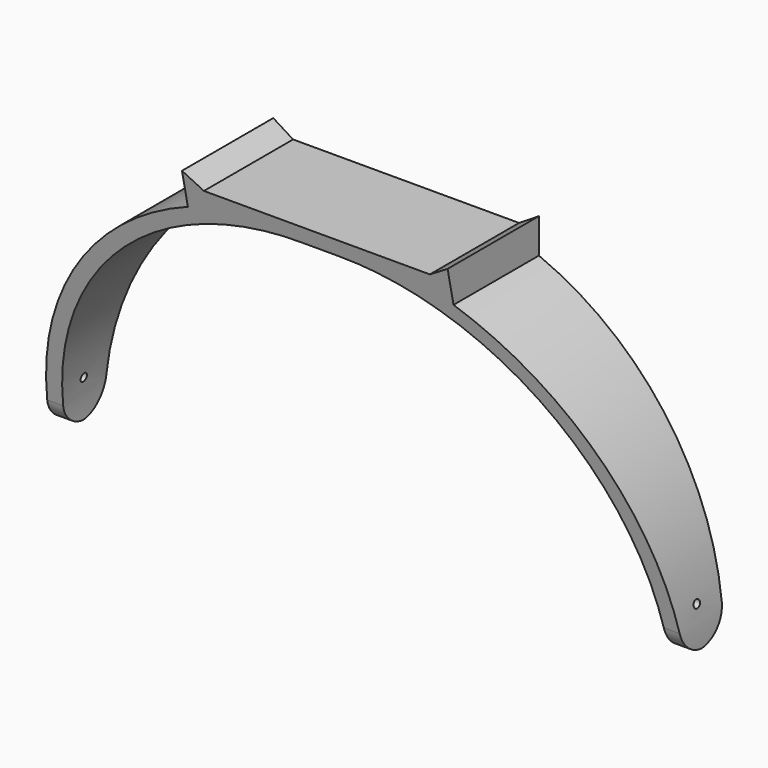
from build123d import *

# Parameters (mm, degrees)
F1_DEPTH      = 25.4
F3_DEPTH      = 40.641
F3_DEPTH_BACK = 40.641
F4_R          = 0.508
F5_DEPTH      = 40.641
F5_DEPTH_BACK = 40.641
F6_T1_DEPTH   = 17.4583858324
F6_T3_DEPTH   = 21.082
F6_T5_DEPTH   = 21.082
F6_T7_DEPTH   = 17.4583858324


# Not quite as in the source:
# - a fillet or chamfer that OpenCascade refuses, or shapes differently, is made with other operations: its cross-section is extruded or revolved along the edge and cut away or added


with BuildPart() as f1:
    # F0 (on Front) → F1 (new body)
    with BuildSketch(Plane.XZ):
        with BuildLine():
            Line((2.54, 0), (0, 0))
            Line((0, 0), (-2.54, 0))
            Line((-2.54, 0), (-14.478, 0))
            Line((-14.478, 0), (-17.018, 0))
            Line((-17.018, 0), (-17.018, -2.8580148686))
            ThreePointArc((-17.018, -2.8580148686), (-34.1882369177, -16.8868177776), (-40.64, -38.1))
            Line((-40.64, -38.1), (-38.608, -38.1))
            ThreePointArc((-38.608, -38.1), (-28.0439273838, -12.5960726162), (-2.54, -2.032))
            Line((-2.54, -2.032), (0, -2.032))
            Line((0, -2.032), (2.54, -2.032))
            ThreePointArc((2.54, -2.032), (28.0439273838, -12.5960726162), (38.608, -38.1))
            Line((38.608, -38.1), (40.64, -38.1))
            ThreePointArc((40.64, -38.1), (34.1882369177, -16.8868177776), (17.018, -2.8580148686))
            Line((17.018, -2.8580148686), (17.018, 0))
            Line((17.018, 0), (14.478, 0))
            Line((14.478, 0), (2.54, 0))
        make_face()
        Polygon((-17.018, 0), (-14.478, 0), (-17.018, 1.5875), align=None)
        Polygon((17.018, 1.5875), (14.478, 0), (17.018, 0), align=None)
    extrude(amount=F1_DEPTH)

    # F2 (on Right) → F3 (cut, two sides)
    with BuildSketch(Plane.YZ) as f3_sk:
        Polygon((-30.48, -50.8), (-3.4853166679, -50.8), (-30.48, 76.2), align=None)
    extrude(amount=-F3_DEPTH, mode=Mode.SUBTRACT)
    extrude(f3_sk.sketch, amount=F3_DEPTH_BACK, mode=Mode.SUBTRACT)

    # F4 (on Right) → F5 (cut, two sides)
    with BuildSketch(Plane.YZ) as f5_sk:
        with Locations((-3.81, -33.02)):
            Circle(F4_R)
    extrude(amount=-F5_DEPTH, mode=Mode.SUBTRACT)
    extrude(f5_sk.sketch, amount=F5_DEPTH_BACK, mode=Mode.SUBTRACT)

    # F6: fillet of radius 3.81 on 4 edges, made by hand

    # F6_s2 → F6_t1 (cut)
    with BuildSketch(Plane.YZ.offset(30.8948070838)):
        with BuildLine():
            ThreePointArc((-6.8262501934, -35.082143542), (-5.4972185245, -37.2509261132), (-3.0995078346, -38.1))
            Line((-3.0995078346, -38.1), (-6.1847850011, -38.1))
            Line((-6.1847850011, -38.1), (-6.8262501934, -35.082143542))
        make_face()
    extrude(amount=F6_T1_DEPTH, mode=Mode.SUBTRACT)

    # F6_s4 → F6_t3 (cut)
    with BuildSketch(Plane.YZ.offset(29.083)):
        with BuildLine():
            ThreePointArc((0, -34.29), (-1.1159231637, -36.9840768363), (-3.81, -38.1))
            Line((-3.81, -38.1), (0, -38.1))
            Line((0, -38.1), (0, -34.29))
        make_face()
    extrude(amount=F6_T3_DEPTH, mode=Mode.SUBTRACT)

    # F6_s6 → F6_t5 (cut)
    with BuildSketch(Plane.YZ.offset(-50.165)):
        with BuildLine():
            ThreePointArc((0, -34.29), (-1.1159231637, -36.9840768363), (-3.81, -38.1))
            Line((-3.81, -38.1), (0, -38.1))
            Line((0, -38.1), (0, -34.29))
        make_face()
    extrude(amount=F6_T5_DEPTH, mode=Mode.SUBTRACT)

    # F6_s8 → F6_t7 (cut)
    with BuildSketch(Plane.YZ.offset(-48.3531929162)):
        with BuildLine():
            ThreePointArc((-6.8262501934, -35.082143542), (-5.4972185245, -37.2509261132), (-3.0995078346, -38.1))
            Line((-3.0995078346, -38.1), (-6.1847850011, -38.1))
            Line((-6.1847850011, -38.1), (-6.8262501934, -35.082143542))
        make_face()
    extrude(amount=F6_T7_DEPTH, mode=Mode.SUBTRACT)


solid = f1.part
